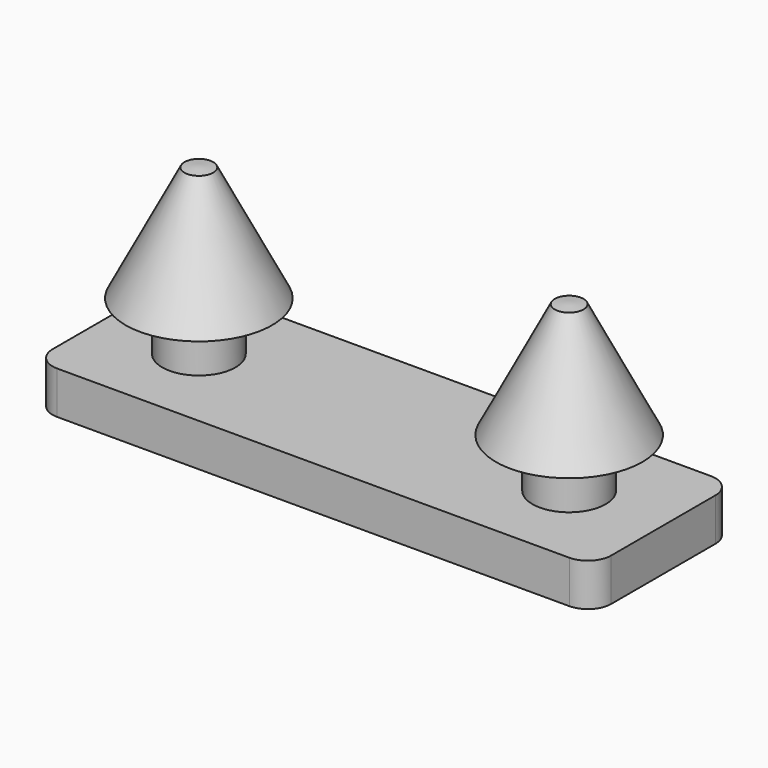
from build123d import *

# Parameters (mm, degrees)
F4_DEPTH = 21
F5_R     = 5
F7_W     = 165.3024330735
F7_H     = 19.5967741311
F8_DEPTH = 19.001
F9_DEPTH = 19.001


# Not quite as in the source:
# - a feature of the source that left no trace in its solid (it failed there, or was rolled back) is left out


with BuildPart() as f1:
    # F0 (on Front) → F1 (revolve)
    with BuildSketch(Plane.XZ):
        Polygon((-47.6422980428, 10.5403326452), (-47.6422980428, 0), (-39.772182703, 0), (-39.772182703, 35.5560481548), (-42.8640134633, 35.2749750018), (-55.5124096572, 10.5403326452), align=None)
    revolve(axis=Axis((-39.772182703, 0, 14.0533037484), (0, 0, 1)))


with BuildPart() as f2_1:
    # F2: instance of F1
    add(f1.part.mirror(Plane.YZ))


with BuildPart() as f4:
    # F3 (on Top) → F4 (new body)
    with BuildSketch(Plane.XY):
        Polygon((-60, 19), (-60, 0), (-60, -19), (60, -19), (60, 19), align=None)
    extrude(amount=-F4_DEPTH)

    # F5
    f5_edges = [f4.edges().sort_by_distance(p)[0] for p in [
        (60, -19, -10.5),
        (-60, -19, -10.5),
        (60, 19, -10.5),
        (-60, 19, -10.5),
    ]]
    fillet(f5_edges, radius=F5_R)

    # F7 (on Front) → F8 (cut, through all)
    with BuildSketch(Plane.XZ):
        with Locations((-2.3588724434, -18.9616940916)):
            Rectangle(F7_W, F7_H)
    extrude(amount=-F8_DEPTH, mode=Mode.SUBTRACT)

    # F9 (cut, through all): a face of the model
    f9_faces = [f4.faces().sort_by_distance(p)[0] for p in [
        (0, 0, -15.081653513),
    ]]
    extrude(f9_faces, amount=-F9_DEPTH, mode=Mode.SUBTRACT)


solid = Compound([f1.part, f2_1.part, f4.part])
